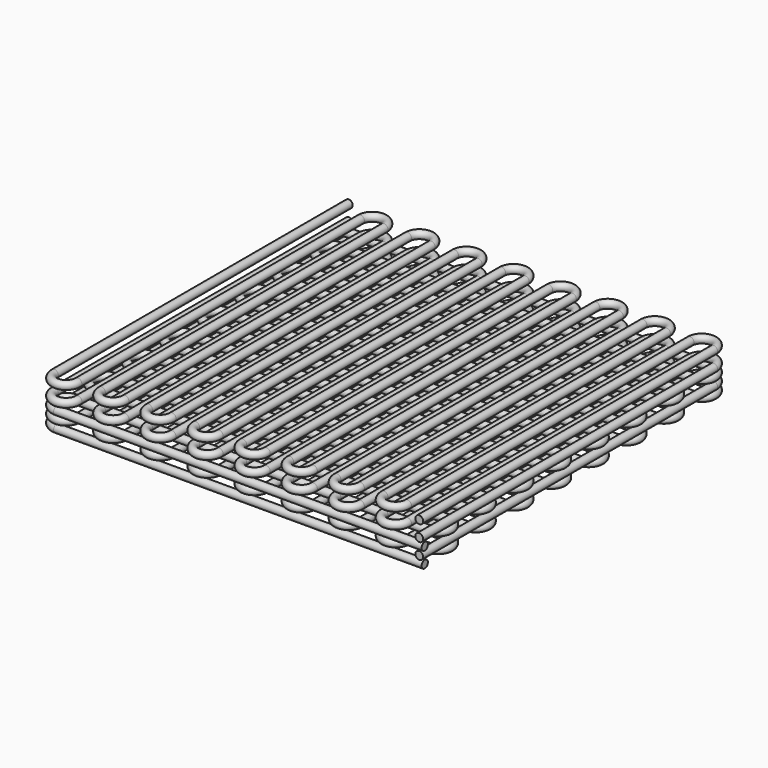
from build123d import *

# Parameters (mm, degrees)
F8_R  = 0.205
F12_R = 0.205
F16_R = 0.205
F20_R = 0.205
F27_R = 0.205


with BuildPart() as f9:
    # F9: sweep along a path in F6
    with BuildLine(Plane.XY.offset(0.615)) as f9_path:
        Line((-10, 9.84), (9.225, 9.84))
        ThreePointArc((9.225, 9.84), (9.84, 9.225), (9.225, 8.61))
        Line((9.225, 8.61), (-9.225, 8.61))
        ThreePointArc((-9.225, 8.61), (-9.84, 7.995), (-9.225, 7.38))
        Line((-9.225, 7.38), (9.225, 7.38))
        ThreePointArc((9.225, 7.38), (9.84, 6.765), (9.225, 6.15))
        Line((9.225, 6.15), (-9.225, 6.15))
        ThreePointArc((-9.225, 6.15), (-9.84, 5.535), (-9.225, 4.92))
        Line((-9.225, 4.92), (9.225, 4.92))
        ThreePointArc((9.225, 4.92), (9.84, 4.305), (9.225, 3.69))
        Line((9.225, 3.69), (-9.225, 3.69))
        ThreePointArc((-9.225, 3.69), (-9.84, 3.075), (-9.225, 2.46))
        Line((-9.225, 2.46), (9.225, 2.46))
        ThreePointArc((9.225, 2.46), (9.84, 1.845), (9.225, 1.23))
        Line((9.225, 1.23), (-9.225, 1.23))
        ThreePointArc((-9.225, 1.23), (-9.84, 0.615), (-9.225, 0))
        Line((-9.225, 0), (9.225, 0))
        ThreePointArc((9.225, 0), (9.84, -0.615), (9.225, -1.23))
        Line((9.225, -1.23), (-9.225, -1.23))
        ThreePointArc((-9.225, -1.23), (-9.84, -1.845), (-9.225, -2.46))
        Line((-9.225, -2.46), (9.225, -2.46))
        ThreePointArc((9.225, -2.46), (9.84, -3.075), (9.225, -3.69))
        Line((9.225, -3.69), (-9.225, -3.69))
        ThreePointArc((-9.225, -3.69), (-9.84, -4.305), (-9.225, -4.92))
        Line((-9.225, -4.92), (9.225, -4.92))
        ThreePointArc((9.225, -4.92), (9.84, -5.535), (9.225, -6.15))
        Line((9.225, -6.15), (-9.225, -6.15))
        ThreePointArc((-9.225, -6.15), (-9.84, -6.765), (-9.225, -7.38))
        Line((-9.225, -7.38), (9.225, -7.38))
        ThreePointArc((9.225, -7.38), (9.84, -7.995), (9.225, -8.61))
        Line((9.225, -8.61), (-9.225, -8.61))
        ThreePointArc((-9.225, -8.61), (-9.84, -9.225), (-9.225, -9.84))
        Line((-9.225, -9.84), (10, -9.84))
    # F8 (on line) → F9 (sweep)
    with BuildSketch(Plane(origin=(-10, 0, 0), x_dir=(0, -1, 0), z_dir=(-1, 0, 0))):
        with Locations((-9.84, 0.615)):
            Circle(F8_R)
    sweep(path=f9_path.line)


with BuildPart() as f13:
    # F13: sweep along a path in F11
    with BuildLine(Plane.XY.offset(1.025)) as f13_path:
        Line((9.84, -10), (9.84, 9.225))
        ThreePointArc((9.84, 9.225), (9.225, 9.84), (8.61, 9.225))
        Line((8.61, 9.225), (8.61, -9.225))
        ThreePointArc((8.61, -9.225), (7.995, -9.84), (7.38, -9.225))
        Line((7.38, -9.225), (7.38, 9.225))
        ThreePointArc((7.38, 9.225), (6.765, 9.84), (6.15, 9.225))
        Line((6.15, 9.225), (6.15, -9.225))
        ThreePointArc((6.15, -9.225), (5.535, -9.84), (4.92, -9.225))
        Line((4.92, -9.225), (4.92, 9.225))
        ThreePointArc((4.92, 9.225), (4.305, 9.84), (3.69, 9.225))
        Line((3.69, 9.225), (3.69, -9.225))
        ThreePointArc((3.69, -9.225), (3.075, -9.84), (2.46, -9.225))
        Line((2.46, -9.225), (2.46, 9.225))
        ThreePointArc((2.46, 9.225), (1.845, 9.84), (1.23, 9.225))
        Line((1.23, 9.225), (1.23, -9.225))
        ThreePointArc((1.23, -9.225), (0.615, -9.84), (0, -9.225))
        Line((0, -9.225), (0, 9.225))
        ThreePointArc((0, 9.225), (-0.615, 9.84), (-1.23, 9.225))
        Line((-1.23, 9.225), (-1.23, -9.225))
        ThreePointArc((-1.23, -9.225), (-1.845, -9.84), (-2.46, -9.225))
        Line((-2.46, -9.225), (-2.46, 9.225))
        ThreePointArc((-2.46, 9.225), (-3.075, 9.84), (-3.69, 9.225))
        Line((-3.69, 9.225), (-3.69, -9.225))
        ThreePointArc((-3.69, -9.225), (-4.305, -9.84), (-4.92, -9.225))
        Line((-4.92, -9.225), (-4.92, 9.225))
        ThreePointArc((-4.92, 9.225), (-5.535, 9.84), (-6.15, 9.225))
        Line((-6.15, 9.225), (-6.15, -9.225))
        ThreePointArc((-6.15, -9.225), (-6.765, -9.84), (-7.38, -9.225))
        Line((-7.38, -9.225), (-7.38, 9.225))
        ThreePointArc((-7.38, 9.225), (-7.995, 9.84), (-8.61, 9.225))
        Line((-8.61, 9.225), (-8.61, -9.225))
        ThreePointArc((-8.61, -9.225), (-9.225, -9.84), (-9.84, -9.225))
        Line((-9.84, -9.225), (-9.84, 10))
    # F12 (on line) → F13 (sweep)
    with BuildSketch(Plane(origin=(0, -10, 0), x_dir=(-1, 0, 0), z_dir=(0, 1, 0))):
        with Locations((-9.84, 1.025)):
            Circle(F12_R)
    sweep(path=f13_path.line)


with BuildPart() as f17:
    # F17: sweep along a path in F15
    with BuildLine(Plane.XY.offset(1.435)) as f17_path:
        Line((-10, 9.84), (9.225, 9.84))
        ThreePointArc((9.225, 9.84), (9.84, 9.225), (9.225, 8.61))
        Line((9.225, 8.61), (-9.225, 8.61))
        ThreePointArc((-9.225, 8.61), (-9.84, 7.995), (-9.225, 7.38))
        Line((-9.225, 7.38), (9.225, 7.38))
        ThreePointArc((9.225, 7.38), (9.84, 6.765), (9.225, 6.15))
        Line((9.225, 6.15), (-9.225, 6.15))
        ThreePointArc((-9.225, 6.15), (-9.84, 5.535), (-9.225, 4.92))
        Line((-9.225, 4.92), (9.225, 4.92))
        ThreePointArc((9.225, 4.92), (9.84, 4.305), (9.225, 3.69))
        Line((9.225, 3.69), (-9.225, 3.69))
        ThreePointArc((-9.225, 3.69), (-9.84, 3.075), (-9.225, 2.46))
        Line((-9.225, 2.46), (9.225, 2.46))
        ThreePointArc((9.225, 2.46), (9.84, 1.845), (9.225, 1.23))
        Line((9.225, 1.23), (-9.225, 1.23))
        ThreePointArc((-9.225, 1.23), (-9.84, 0.615), (-9.225, 0))
        Line((-9.225, 0), (9.225, 0))
        ThreePointArc((9.225, 0), (9.84, -0.615), (9.225, -1.23))
        Line((9.225, -1.23), (-9.225, -1.23))
        ThreePointArc((-9.225, -1.23), (-9.84, -1.845), (-9.225, -2.46))
        Line((-9.225, -2.46), (9.225, -2.46))
        ThreePointArc((9.225, -2.46), (9.84, -3.075), (9.225, -3.69))
        Line((9.225, -3.69), (-9.225, -3.69))
        ThreePointArc((-9.225, -3.69), (-9.84, -4.305), (-9.225, -4.92))
        Line((-9.225, -4.92), (9.225, -4.92))
        ThreePointArc((9.225, -4.92), (9.84, -5.535), (9.225, -6.15))
        Line((9.225, -6.15), (-9.225, -6.15))
        ThreePointArc((-9.225, -6.15), (-9.84, -6.765), (-9.225, -7.38))
        Line((-9.225, -7.38), (9.225, -7.38))
        ThreePointArc((9.225, -7.38), (9.84, -7.995), (9.225, -8.61))
        Line((9.225, -8.61), (-9.225, -8.61))
        ThreePointArc((-9.225, -8.61), (-9.84, -9.225), (-9.225, -9.84))
        Line((-9.225, -9.84), (10, -9.84))
    # F16 (on line) → F17 (sweep)
    with BuildSketch(Plane(origin=(-10, 0, 0), x_dir=(0, -1, 0), z_dir=(-1, 0, 0))):
        with Locations((-9.84, 1.435)):
            Circle(F16_R)
    sweep(path=f17_path.line)


with BuildPart() as f21:
    # F21: sweep along a path in F19
    with BuildLine(Plane.XY.offset(1.845)) as f21_path:
        Line((9.84, -10), (9.84, 9.225))
        ThreePointArc((9.84, 9.225), (9.225, 9.84), (8.61, 9.225))
        Line((8.61, 9.225), (8.61, -9.225))
        ThreePointArc((8.61, -9.225), (7.995, -9.84), (7.38, -9.225))
        Line((7.38, -9.225), (7.38, 9.225))
        ThreePointArc((7.38, 9.225), (6.765, 9.84), (6.15, 9.225))
        Line((6.15, 9.225), (6.15, -9.225))
        ThreePointArc((6.15, -9.225), (5.535, -9.84), (4.92, -9.225))
        Line((4.92, -9.225), (4.92, 9.225))
        ThreePointArc((4.92, 9.225), (4.305, 9.84), (3.69, 9.225))
        Line((3.69, 9.225), (3.69, -9.225))
        ThreePointArc((3.69, -9.225), (3.075, -9.84), (2.46, -9.225))
        Line((2.46, -9.225), (2.46, 9.225))
        ThreePointArc((2.46, 9.225), (1.845, 9.84), (1.23, 9.225))
        Line((1.23, 9.225), (1.23, -9.225))
        ThreePointArc((1.23, -9.225), (0.615, -9.84), (0, -9.225))
        Line((0, -9.225), (0, 9.225))
        ThreePointArc((0, 9.225), (-0.615, 9.84), (-1.23, 9.225))
        Line((-1.23, 9.225), (-1.23, -9.225))
        ThreePointArc((-1.23, -9.225), (-1.845, -9.84), (-2.46, -9.225))
        Line((-2.46, -9.225), (-2.46, 9.225))
        ThreePointArc((-2.46, 9.225), (-3.075, 9.84), (-3.69, 9.225))
        Line((-3.69, 9.225), (-3.69, -9.225))
        ThreePointArc((-3.69, -9.225), (-4.305, -9.84), (-4.92, -9.225))
        Line((-4.92, -9.225), (-4.92, 9.225))
        ThreePointArc((-4.92, 9.225), (-5.535, 9.84), (-6.15, 9.225))
        Line((-6.15, 9.225), (-6.15, -9.225))
        ThreePointArc((-6.15, -9.225), (-6.765, -9.84), (-7.38, -9.225))
        Line((-7.38, -9.225), (-7.38, 9.225))
        ThreePointArc((-7.38, 9.225), (-7.995, 9.84), (-8.61, 9.225))
        Line((-8.61, 9.225), (-8.61, -9.225))
        ThreePointArc((-8.61, -9.225), (-9.225, -9.84), (-9.84, -9.225))
        Line((-9.84, -9.225), (-9.84, 10))
    # F20 (on line) → F21 (sweep)
    with BuildSketch(Plane(origin=(0, -10, 0), x_dir=(-1, 0, 0), z_dir=(0, 1, 0))):
        with Locations((-9.84, 1.845)):
            Circle(F20_R)
    sweep(path=f21_path.line)


with BuildPart() as f28:
    # F28: sweep along a path in F26
    with BuildLine(Plane.XY.offset(2.665)) as f28_path:
        Line((9.84, -10), (9.84, 9.225))
        ThreePointArc((9.84, 9.225), (9.225, 9.84), (8.61, 9.225))
        Line((8.61, 9.225), (8.61, -9.225))
        ThreePointArc((8.61, -9.225), (7.995, -9.84), (7.38, -9.225))
        Line((7.38, -9.225), (7.38, 9.225))
        ThreePointArc((7.38, 9.225), (6.765, 9.84), (6.15, 9.225))
        Line((6.15, 9.225), (6.15, -9.225))
        ThreePointArc((6.15, -9.225), (5.535, -9.84), (4.92, -9.225))
        Line((4.92, -9.225), (4.92, 9.225))
        ThreePointArc((4.92, 9.225), (4.305, 9.84), (3.69, 9.225))
        Line((3.69, 9.225), (3.69, -9.225))
        ThreePointArc((3.69, -9.225), (3.075, -9.84), (2.46, -9.225))
        Line((2.46, -9.225), (2.46, 9.225))
        ThreePointArc((2.46, 9.225), (1.845, 9.84), (1.23, 9.225))
        Line((1.23, 9.225), (1.23, -9.225))
        ThreePointArc((1.23, -9.225), (0.615, -9.84), (0, -9.225))
        Line((0, -9.225), (0, 9.225))
        ThreePointArc((0, 9.225), (-0.615, 9.84), (-1.23, 9.225))
        Line((-1.23, 9.225), (-1.23, -9.225))
        ThreePointArc((-1.23, -9.225), (-1.845, -9.84), (-2.46, -9.225))
        Line((-2.46, -9.225), (-2.46, 9.225))
        ThreePointArc((-2.46, 9.225), (-3.075, 9.84), (-3.69, 9.225))
        Line((-3.69, 9.225), (-3.69, -9.225))
        ThreePointArc((-3.69, -9.225), (-4.305, -9.84), (-4.92, -9.225))
        Line((-4.92, -9.225), (-4.92, 9.225))
        ThreePointArc((-4.92, 9.225), (-5.535, 9.84), (-6.15, 9.225))
        Line((-6.15, 9.225), (-6.15, -9.225))
        ThreePointArc((-6.15, -9.225), (-6.765, -9.84), (-7.38, -9.225))
        Line((-7.38, -9.225), (-7.38, 9.225))
        ThreePointArc((-7.38, 9.225), (-7.995, 9.84), (-8.61, 9.225))
        Line((-8.61, 9.225), (-8.61, -9.225))
        ThreePointArc((-8.61, -9.225), (-9.225, -9.84), (-9.84, -9.225))
        Line((-9.84, -9.225), (-9.84, 10))
    # F27 (on line) → F28 (sweep)
    with BuildSketch(Plane(origin=(0, -10, 0), x_dir=(-1, 0, 0), z_dir=(0, 1, 0))):
        with Locations((-9.84, 2.665)):
            Circle(F27_R)
    sweep(path=f28_path.line)


solid = Compound([f9.part, f13.part, f17.part, f21.part, f28.part])
